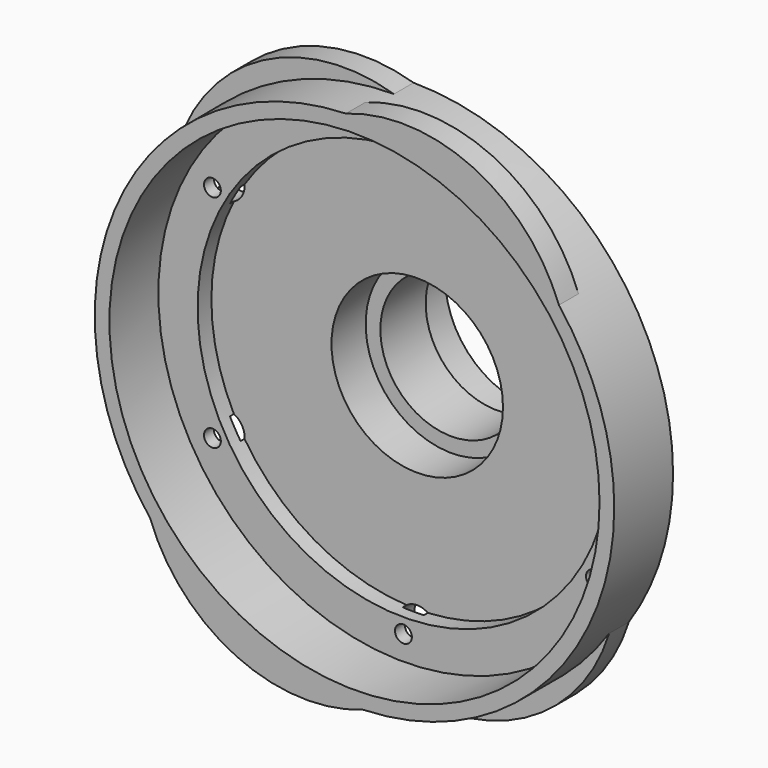
from build123d import *

# Parameters (mm, degrees)
F0_R          = 33.655
F1_DEPTH      = 28.575
F2_R          = 43.8466719597
F2_R_2        = 12.7
F3_DEPTH      = 15.875
F4_R          = 31.75
F5_DEPTH      = 7.9248
F6_R          = 26.67
F7_DEPTH      = 2.2352
F8_R          = 11.10996
F9_DEPTH      = 5.5372
F10_R         = 9.2075
F11_DEPTH     = 25.4
F12_R         = 11.10996
F13_DEPTH     = 5.5372
F14_R         = 43.7649146766
F14_R_2       = 29.21
F15_DEPTH     = 3.175
F16_R         = 1.0922
F17_DEPTH     = 25.4
F18_R         = 2.3749
F19_DEPTH     = 3.175
F20_T4_ANGLE  = 58.3951667525
F20_S5_R      = 2.3749
F20_T6_DEPTH  = 18
F20_S7_R      = 2.3749
F20_T8_DEPTH  = 18
F20_T12_ANGLE = 58.3951667525
F20_S13_R     = 2.3749
F20_T14_DEPTH = 18
F20_S15_R     = 2.3749
F20_T16_DEPTH = 18
F20_T20_ANGLE = 58.3951667525
F20_S21_R     = 2.3749
F20_T22_DEPTH = 18
F20_S23_R     = 2.3749
F20_T24_DEPTH = 18
F20_T28_ANGLE = 58.3951667525
F20_S29_R     = 2.3749
F20_T30_DEPTH = 18
F20_S31_R     = 2.3749
F20_T32_DEPTH = 18
F20_T36_ANGLE = 58.3951667525
F20_S37_R     = 2.3749
F20_T38_DEPTH = 18
F20_S39_R     = 2.3749
F20_T40_DEPTH = 18
F20_T44_ANGLE = 58.3951667525
F20_S45_R     = 2.3749
F20_T46_DEPTH = 18
F20_S47_R     = 2.3749
F20_T48_DEPTH = 18
F20_T50_ANGLE = 58.3951667525
F20_T52_ANGLE = 58.3951667525
F20_T54_ANGLE = 58.3951667525
F20_T56_ANGLE = 58.3951667525
F20_T58_ANGLE = 58.3951667525
F20_T60_ANGLE = 58.3951667525
F22_DEPTH     = 3.175
F24_DEPTH     = 3.175


# Not quite as in the source:
# - a fillet or chamfer that OpenCascade refuses, or shapes differently, is made with other operations: its cross-section is extruded or revolved along the edge and cut away or added


with BuildPart() as f1:
    # F0 (on Front) → F1 (new body)
    with BuildSketch(Plane.XZ):
        Circle(F0_R)
    extrude(amount=F1_DEPTH)

    # F2 (on face) → F3 (cut)
    with BuildSketch(Plane(origin=(0, 0, 0), x_dir=(-1, 0, 0), z_dir=(0, 1, 0))):
        Circle(F2_R)
        Circle(F2_R_2, mode=Mode.SUBTRACT)
    extrude(amount=-F3_DEPTH, mode=Mode.SUBTRACT)

    # F4 (on face) → F5 (cut)
    with BuildSketch(Plane.XZ.offset(28.575)):
        Circle(F4_R)
    extrude(amount=-F5_DEPTH, mode=Mode.SUBTRACT)

    # F6 (on face) → F7 (cut)
    with BuildSketch(Plane.XZ.offset(20.6502)):
        Circle(F6_R)
    extrude(amount=-F7_DEPTH, mode=Mode.SUBTRACT)

    # F8 (on face) → F9 (cut)
    with BuildSketch(Plane.XZ.offset(18.415)):
        Circle(F8_R)
    extrude(amount=-F9_DEPTH, mode=Mode.SUBTRACT)

    # F10 (on face) → F11 (cut)
    with BuildSketch(Plane.XZ.offset(12.8778)):
        Circle(F10_R)
    extrude(amount=-F11_DEPTH, mode=Mode.SUBTRACT)

    # F12 (on face) → F13 (cut)
    with BuildSketch(Plane(origin=(0, 0, 0), x_dir=(-1, 0, 0), z_dir=(0, 1, 0))):
        Circle(F12_R)
    extrude(amount=-F13_DEPTH, mode=Mode.SUBTRACT)

    # F14 (on face) → F15 (cut)
    with BuildSketch(Plane(origin=(0, -15.875, 0), x_dir=(-1, 0, 0), z_dir=(0, 1, 0))):
        Circle(F14_R)
        Circle(F14_R_2, mode=Mode.SUBTRACT)
    extrude(amount=-F15_DEPTH, mode=Mode.SUBTRACT)

    # F16 (on face) → F17 (cut)
    with BuildSketch(Plane.XZ.offset(20.6502)):
        with Locations((0, 28.575)):
            Circle(F16_R)
        with Locations((-24.7466759131, 14.2875)):
            Circle(F16_R)
        with Locations((-24.7466759131, -14.2875)):
            Circle(F16_R)
        with Locations((0, -28.575)):
            Circle(F16_R)
        with Locations((24.7466759131, -14.2875)):
            Circle(F16_R)
        with Locations((24.7466759131, 14.2875)):
            Circle(F16_R)
    extrude(amount=-F17_DEPTH, mode=Mode.SUBTRACT)

    # F18 (on face) → F19 (cut)
    with BuildSketch(Plane(origin=(0, -15.875, 0), x_dir=(-1, 0, 0), z_dir=(0, 1, 0))):
        with Locations((0, 28.575)):
            Circle(F18_R)
        with Locations((-24.7466759131, 14.2875)):
            Circle(F18_R)
        with Locations((-24.7466759131, -14.2875)):
            Circle(F18_R)
        with Locations((0, -28.575)):
            Circle(F18_R)
        with Locations((24.7466759131, -14.2875)):
            Circle(F18_R)
        with Locations((24.7466759131, 14.2875)):
            Circle(F18_R)
    extrude(amount=-F19_DEPTH, mode=Mode.SUBTRACT)

    # F20: fillet of radius 0.762 on 12 edges, made by hand


with BuildPart() as f20_tool2:
    # F20_s3 → F20_t4 (revolve)
    with BuildSketch(Plane(origin=(0, 0, 0), x_dir=(0, 1, 0), z_dir=(-0.9999019342, 0, 0.0140043543))):
        with BuildLine():
            ThreePointArc((-18.288, -29.21), (-18.8268153673, -29.4331846327), (-19.05, -29.972))
            Line((-19.05, -29.972), (-19.05, -29.21))
            Line((-19.05, -29.21), (-18.288, -29.21))
        make_face()
    revolve(axis=Axis((0, -19.05, 0), (0, 1, 0)), revolution_arc=F20_T4_ANGLE)

    # F20_s5 → F20_t6 (cut, symmetric)
    with BuildSketch(Plane.XZ.offset(18.4)):
        with Locations((24.7466759131, 14.2875)):
            Circle(F20_S5_R)
    extrude(amount=F20_T6_DEPTH, both=True, mode=Mode.SUBTRACT)

    # F20_s7 → F20_t8 (cut, symmetric)
    with BuildSketch(Plane.XZ.offset(18.4)):
        with Locations((0, 28.575)):
            Circle(F20_S7_R)
    extrude(amount=F20_T8_DEPTH, both=True, mode=Mode.SUBTRACT)


with BuildPart() as f1_1:
    add(f1.part)

    # F20_t1: union F20_tool2
    add(f20_tool2.part)


with BuildPart() as f20_tool10:
    # F20_s11 → F20_t12 (revolve)
    with BuildSketch(Plane(origin=(0, 0, 0), x_dir=(0, 1, 0), z_dir=(-0.4878228406, 0, 0.8729426535))):
        with BuildLine():
            ThreePointArc((-18.288, -29.21), (-18.8268153673, -29.4331846327), (-19.05, -29.972))
            Line((-19.05, -29.972), (-19.05, -29.21))
            Line((-19.05, -29.21), (-18.288, -29.21))
        make_face()
    revolve(axis=Axis((0, -19.05, 0), (0, 1, 0)), revolution_arc=F20_T12_ANGLE)

    # F20_s13 → F20_t14 (cut, symmetric)
    with BuildSketch(Plane.XZ.offset(18.4)):
        with Locations((24.7466759131, 14.2875)):
            Circle(F20_S13_R)
    extrude(amount=F20_T14_DEPTH, both=True, mode=Mode.SUBTRACT)

    # F20_s15 → F20_t16 (cut, symmetric)
    with BuildSketch(Plane.XZ.offset(18.4)):
        with Locations((24.7466759131, -14.2875)):
            Circle(F20_S15_R)
    extrude(amount=F20_T16_DEPTH, both=True, mode=Mode.SUBTRACT)


with BuildPart() as f1_2:
    add(f1_1.part)

    # F20_t9: union F20_tool10
    add(f20_tool10.part)


with BuildPart() as f20_tool18:
    # F20_s19 → F20_t20 (revolve)
    with BuildSketch(Plane(origin=(0, 0, 0), x_dir=(0, 1, 0), z_dir=(0.5120790937, 0, 0.8589382992))):
        with BuildLine():
            ThreePointArc((-18.288, -29.21), (-18.8268153673, -29.4331846327), (-19.05, -29.972))
            Line((-19.05, -29.972), (-19.05, -29.21))
            Line((-19.05, -29.21), (-18.288, -29.21))
        make_face()
    revolve(axis=Axis((0, -19.05, 0), (0, 1, 0)), revolution_arc=F20_T20_ANGLE)

    # F20_s21 → F20_t22 (cut, symmetric)
    with BuildSketch(Plane.XZ.offset(18.4)):
        with Locations((24.7466759131, -14.2875)):
            Circle(F20_S21_R)
    extrude(amount=F20_T22_DEPTH, both=True, mode=Mode.SUBTRACT)

    # F20_s23 → F20_t24 (cut, symmetric)
    with BuildSketch(Plane.XZ.offset(18.4)):
        with Locations((0, -28.575)):
            Circle(F20_S23_R)
    extrude(amount=F20_T24_DEPTH, both=True, mode=Mode.SUBTRACT)


with BuildPart() as f1_3:
    add(f1_2.part)

    # F20_t17: union F20_tool18
    add(f20_tool18.part)


with BuildPart() as f20_tool26:
    # F20_s27 → F20_t28 (revolve)
    with BuildSketch(Plane(origin=(0, 0, 0), x_dir=(0, 1, 0), z_dir=(0.4878228406, 0, 0.8729426535))):
        with BuildLine():
            ThreePointArc((-18.288, 29.21), (-18.8268153673, 29.4331846327), (-19.05, 29.972))
            Line((-19.05, 29.972), (-19.05, 29.21))
            Line((-19.05, 29.21), (-18.288, 29.21))
        make_face()
    revolve(axis=Axis((0, -19.05, 0), (0, -1, 0)), revolution_arc=F20_T28_ANGLE)

    # F20_s29 → F20_t30 (cut, symmetric)
    with BuildSketch(Plane.XZ.offset(18.4)):
        with Locations((-24.7466759131, 14.2875)):
            Circle(F20_S29_R)
    extrude(amount=F20_T30_DEPTH, both=True, mode=Mode.SUBTRACT)

    # F20_s31 → F20_t32 (cut, symmetric)
    with BuildSketch(Plane.XZ.offset(18.4)):
        with Locations((-24.7466759131, -14.2875)):
            Circle(F20_S31_R)
    extrude(amount=F20_T32_DEPTH, both=True, mode=Mode.SUBTRACT)


with BuildPart() as f1_4:
    add(f1_3.part)

    # F20_t25: union F20_tool26
    add(f20_tool26.part)


with BuildPart() as f20_tool34:
    # F20_s35 → F20_t36 (revolve)
    with BuildSketch(Plane(origin=(0, 0, 0), x_dir=(0, 1, 0), z_dir=(-0.5120790937, 0, -0.8589382992))):
        with BuildLine():
            ThreePointArc((-18.288, -29.21), (-18.8268153673, -29.4331846327), (-19.05, -29.972))
            Line((-19.05, -29.972), (-19.05, -29.21))
            Line((-19.05, -29.21), (-18.288, -29.21))
        make_face()
    revolve(axis=Axis((0, -19.05, 0), (0, 1, 0)), revolution_arc=F20_T36_ANGLE)

    # F20_s37 → F20_t38 (cut, symmetric)
    with BuildSketch(Plane.XZ.offset(18.4)):
        with Locations((0, 28.575)):
            Circle(F20_S37_R)
    extrude(amount=F20_T38_DEPTH, both=True, mode=Mode.SUBTRACT)

    # F20_s39 → F20_t40 (cut, symmetric)
    with BuildSketch(Plane.XZ.offset(18.4)):
        with Locations((-24.7466759131, 14.2875)):
            Circle(F20_S39_R)
    extrude(amount=F20_T40_DEPTH, both=True, mode=Mode.SUBTRACT)


with BuildPart() as f1_5:
    add(f1_4.part)

    # F20_t33: union F20_tool34
    add(f20_tool34.part)


with BuildPart() as f20_tool42:
    # F20_s43 → F20_t44 (revolve)
    with BuildSketch(Plane(origin=(0, 0, 0), x_dir=(0, 1, 0), z_dir=(0.9999019342, 0, -0.0140043543))):
        with BuildLine():
            ThreePointArc((-18.288, -29.21), (-18.8268153673, -29.4331846327), (-19.05, -29.972))
            Line((-19.05, -29.972), (-19.05, -29.21))
            Line((-19.05, -29.21), (-18.288, -29.21))
        make_face()
    revolve(axis=Axis((0, -19.05, 0), (0, 1, 0)), revolution_arc=F20_T44_ANGLE)

    # F20_s45 → F20_t46 (cut, symmetric)
    with BuildSketch(Plane.XZ.offset(18.4)):
        with Locations((0, -28.575)):
            Circle(F20_S45_R)
    extrude(amount=F20_T46_DEPTH, both=True, mode=Mode.SUBTRACT)

    # F20_s47 → F20_t48 (cut, symmetric)
    with BuildSketch(Plane.XZ.offset(18.4)):
        with Locations((-24.7466759131, -14.2875)):
            Circle(F20_S47_R)
    extrude(amount=F20_T48_DEPTH, both=True, mode=Mode.SUBTRACT)


with BuildPart() as f1_6:
    add(f1_5.part)

    # F20_t41: union F20_tool42
    add(f20_tool42.part)

    # F20_s49 → F20_t50 (revolve, cut)
    with BuildSketch(Plane(origin=(0, 0, 0), x_dir=(0, 1, 0), z_dir=(0.9999019342, 0, -0.0140043543))):
        with BuildLine():
            ThreePointArc((-15.875, -28.448), (-16.0981846327, -28.9868153673), (-16.637, -29.21))
            Line((-16.637, -29.21), (-15.875, -29.21))
            Line((-15.875, -29.21), (-15.875, -28.448))
        make_face()
    revolve(axis=Axis((0, -15.875, 0), (0, 1, 0)), revolution_arc=F20_T50_ANGLE, mode=Mode.SUBTRACT)

    # F20_s51 → F20_t52 (revolve, cut)
    with BuildSketch(Plane(origin=(0, 0, 0), x_dir=(0, 1, 0), z_dir=(0.4878228406, 0, 0.8729426535))):
        with BuildLine():
            ThreePointArc((-15.875, 28.448), (-16.0981846327, 28.9868153673), (-16.637, 29.21))
            Line((-16.637, 29.21), (-15.875, 29.21))
            Line((-15.875, 29.21), (-15.875, 28.448))
        make_face()
    revolve(axis=Axis((0, -15.875, 0), (0, -1, 0)), revolution_arc=F20_T52_ANGLE, mode=Mode.SUBTRACT)

    # F20_s53 → F20_t54 (revolve, cut)
    with BuildSketch(Plane(origin=(0, 0, 0), x_dir=(0, 1, 0), z_dir=(0.5120790937, 0, 0.8589382992))):
        with BuildLine():
            ThreePointArc((-15.875, -28.448), (-16.0981846327, -28.9868153673), (-16.637, -29.21))
            Line((-16.637, -29.21), (-15.875, -29.21))
            Line((-15.875, -29.21), (-15.875, -28.448))
        make_face()
    revolve(axis=Axis((0, -15.875, 0), (0, 1, 0)), revolution_arc=F20_T54_ANGLE, mode=Mode.SUBTRACT)

    # F20_s55 → F20_t56 (revolve, cut)
    with BuildSketch(Plane(origin=(0, 0, 0), x_dir=(0, 1, 0), z_dir=(-0.4878228406, 0, 0.8729426535))):
        with BuildLine():
            ThreePointArc((-16.637, -29.21), (-16.0981846327, -28.9868153673), (-15.875, -28.448))
            Line((-15.875, -28.448), (-15.875, -29.21))
            Line((-15.875, -29.21), (-16.637, -29.21))
        make_face()
    revolve(axis=Axis((0, -15.875, 0), (0, 1, 0)), revolution_arc=F20_T56_ANGLE, mode=Mode.SUBTRACT)

    # F20_s57 → F20_t58 (revolve, cut)
    with BuildSketch(Plane(origin=(0, 0, 0), x_dir=(0, 1, 0), z_dir=(-0.9999019342, 0, 0.0140043543))):
        with BuildLine():
            ThreePointArc((-15.875, -28.448), (-16.0981846327, -28.9868153673), (-16.637, -29.21))
            Line((-16.637, -29.21), (-15.875, -29.21))
            Line((-15.875, -29.21), (-15.875, -28.448))
        make_face()
    revolve(axis=Axis((0, -15.875, 0), (0, 1, 0)), revolution_arc=F20_T58_ANGLE, mode=Mode.SUBTRACT)

    # F20_s59 → F20_t60 (revolve, cut)
    with BuildSketch(Plane(origin=(0, 0, 0), x_dir=(0, 1, 0), z_dir=(-0.5120790937, 0, -0.8589382992))):
        with BuildLine():
            ThreePointArc((-15.875, -28.448), (-16.0981846327, -28.9868153673), (-16.637, -29.21))
            Line((-16.637, -29.21), (-15.875, -29.21))
            Line((-15.875, -29.21), (-15.875, -28.448))
        make_face()
    revolve(axis=Axis((0, -15.875, 0), (0, 1, 0)), revolution_arc=F20_T60_ANGLE, mode=Mode.SUBTRACT)

    # F21 (on face) → F22 (join)
    with BuildSketch(Plane.XZ.offset(28.575)):
        with BuildLine():
            ThreePointArc((-3.6870200555, 32.5269122703), (13.8344986129, 29.6681780172), (27.2870312048, 18.0834749636))
            ThreePointArc((27.2870312048, 18.0834749636), (15.32595948, 32.8666261683), (-3.6870200555, 32.5269122703))
        make_face()
        with BuildLine():
            ThreePointArc((-27.2870312048, -18.0834749636), (-15.32595948, -32.8666261683), (3.6870200555, -32.5269122703))
            ThreePointArc((3.6870200555, -32.5269122703), (-13.8344986129, -29.6681780172), (-27.2870312048, -18.0834749636))
        make_face()
    extrude(amount=-F22_DEPTH)

    # F23 (on face) → F24 (join)
    with BuildSketch(Plane(origin=(0, -19.05, 0), x_dir=(-1, 0, 0), z_dir=(0, 1, 0))):
        with BuildLine():
            ThreePointArc((-2.9261285428, 32.567453848), (15.351083205, 28.8711884554), (28.6359131983, 15.7856185718))
            ThreePointArc((28.6359131983, 15.7856185718), (16.9965559886, 31.9658726674), (-2.9261285428, 32.567453848))
        make_face()
        with BuildLine():
            ThreePointArc((-28.6359131983, -15.7856185718), (-16.9965559886, -31.9658726674), (2.9261285428, -32.567453848))
            ThreePointArc((2.9261285428, -32.567453848), (-15.351083205, -28.8711884554), (-28.6359131983, -15.7856185718))
        make_face()
    extrude(amount=-F24_DEPTH)


solid = f1_6.part
